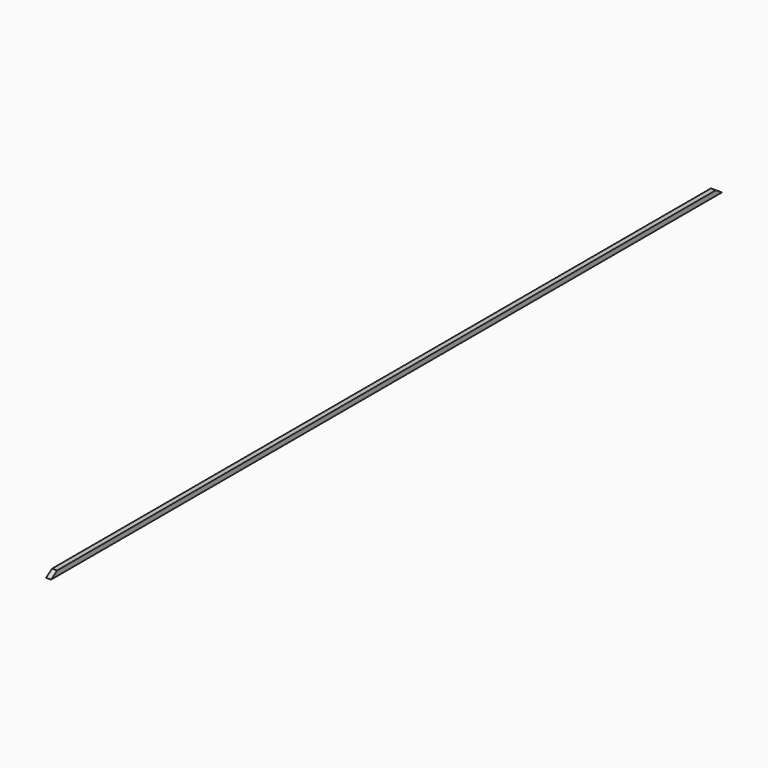
from build123d import *

# Parameters (mm, degrees)
F1_DEPTH = 3.175


# Not quite as in the source:
# - a feature names something its author has since deleted; it is built from what else it names


with BuildPart() as f1:
    # F0 (on Right) → F1 (new body)
    with BuildSketch(Plane.YZ):
        Polygon((-269.230722746, 0), (264.16, 0), (259.344988627, 3.175), (-264.415711373, 3.175), align=None)
    extrude(amount=F1_DEPTH)


solid = f1.part
